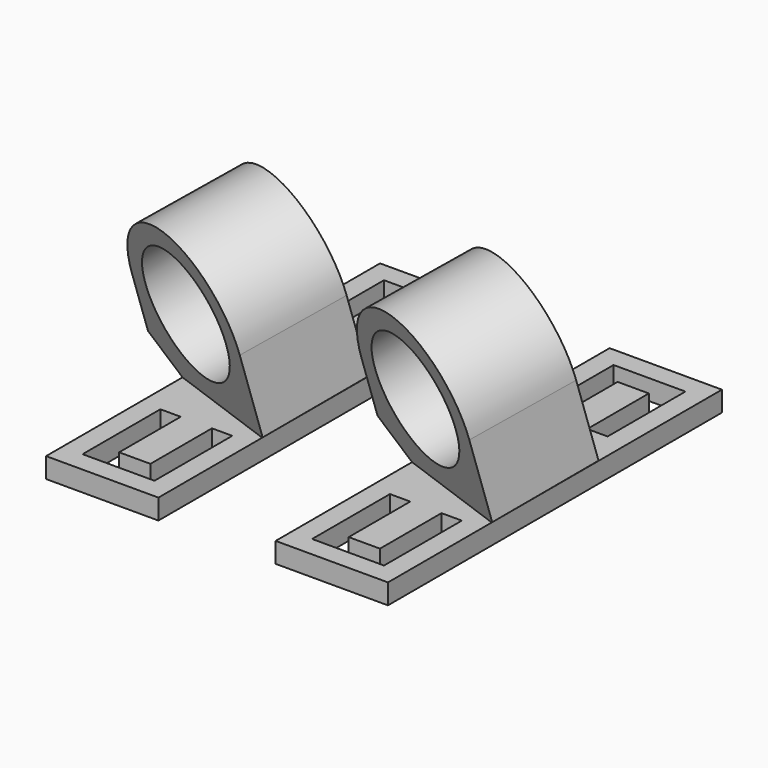
from build123d import *

# Parameters (mm, degrees)
F0_W      = 11.11
F0_H      = 2
F1_DEPTH  = 20.64
F0_R      = 6
F2_DEPTH  = 5
F3_ANGLE  = 15
F4_ANGLE  = -20
F5_REACH  = 31.3423506364
F6_DEPTH  = 6.9
F7_DEPTH  = 25
F11_DEPTH = 25
F12_DEPTH = 31
F15_DEPTH = 25


with BuildPart() as f1:
    # F0 (on Front) → F1 (new body, symmetric)
    with BuildSketch(Plane.XZ):
        with Locations((-58.071229763, 1)):
            Rectangle(F0_W, F0_H)
    extrude(amount=F1_DEPTH, both=True)


with BuildPart() as f2:
    # F0 (on Front) → F2 (new body, symmetric)
    with BuildSketch(Plane.XZ):
        with BuildLine():
            ThreePointArc((-50.071229763, 11.4522753283), (-58.071229763, 19.4522753283), (-66.071229763, 11.4522753283))
            ThreePointArc((-66.071229763, 11.4522753283), (-58.071229763, 3.4522753283), (-50.071229763, 11.4522753283))
        make_face()
        with Locations((-58.071229763, 11.4522753283)):
            Circle(F0_R, mode=Mode.SUBTRACT)
        with BuildLine():
            Line((-66.071229763, 2), (-63.626229763, 2))
            Line((-63.626229763, 2), (-52.516229763, 2))
            Line((-52.516229763, 2), (-50.071229763, 2))
            Line((-50.071229763, 2), (-50.071229763, 11.4522753283))
            ThreePointArc((-50.071229763, 11.4522753283), (-58.071229763, 3.4522753283), (-66.071229763, 11.4522753283))
            Line((-66.071229763, 11.4522753283), (-66.071229763, 2))
        make_face()
    extrude(amount=F2_DEPTH, both=True)


with BuildPart() as f2_1:
    # F3: moved
    add(f2.part.rotate(Axis((-58.071229763, 0, 1), (1, 0, 0)), F3_ANGLE))


with BuildPart() as f2_2:
    # F4: moved
    add(f2_1.part.rotate(Axis((-58.071229763, 0, 1), (0, 0, 1)), F4_ANGLE))


with BuildPart() as f5:
    f5_end = Plane(origin=(-58.071229763, 0, 0), x_dir=(-1, 0, 0), z_dir=(0, 0, -1))
    # F2_face (on face) → F5 (new body, up to a plane its end follows)
    with BuildSketch(Plane(origin=(-58.1597510899, -0.2432103468, 1.9659258263), x_dir=(1, 0, 0), z_dir=(0.0885213269, 0.2432103468, -0.9659258263))):
        Polygon((-9.2055096516, 2.0636356397), (-5.8888283999, -7.3703256425), (9.2055096516, -2.0636356397), (5.8888283999, 7.3703256425), align=None)
    f5_long = extrude(amount=F5_REACH, mode=Mode.PRIVATE)
    add(split(f5_long, bisect_by=f5_end, keep=Keep.BOTTOM, mode=Mode.PRIVATE))


with BuildPart() as f6_tool:
    # F6 (cut): a face of the model
    f6_faces = [f1.part.faces().sort_by_distance(p)[0] for p in [
        (-63.626229763, 0, 1),
    ]]
    extrude(f6_faces, amount=F6_DEPTH)


with BuildPart() as f2_3:
    add(f2_2.part)

    # F6: cut by f6_tool
    add(f6_tool.part, mode=Mode.SUBTRACT)


with BuildPart() as f5_1:
    add(f5.part)

    # F6: cut by f6_tool
    add(f6_tool.part, mode=Mode.SUBTRACT)


with BuildPart() as f7_tool:
    # F7 (cut): a face of the model
    f7_faces = [f1.part.faces().sort_by_distance(p)[0] for p in [
        (-52.516229763, 0, 1),
    ]]
    extrude(f7_faces, amount=F7_DEPTH)


with BuildPart() as f2_4:
    add(f2_3.part)

    # F7: cut by f7_tool
    add(f7_tool.part, mode=Mode.SUBTRACT)


with BuildPart() as f5_2:
    add(f5_1.part)

    # F7: cut by f7_tool
    add(f7_tool.part, mode=Mode.SUBTRACT)


with BuildPart() as f1_1:
    add(f1.part)

    # F8: union F2, F5
    add(f2_4.part)
    add(f5_2.part)


with BuildPart() as f9_1:
    # F9: copy of F1
    add(f1_1.part.moved(Location((28.1, 0, 0))))


with BuildPart() as f1_2:
    add(f1_1.part)

    # F10 (on face) → F11 (cut)
    with BuildSketch(Plane.XZ.offset(20.64)):
        Polygon((-47.5953929126, 6.1317714863), (-52.516229763, 2), (-52.516229763, 0), (-47.5953929126, 0), align=None)
        Polygon((-63.626229763, 0), (-63.626229763, 2), (-68.9108520746, 5.1364828832), (-68.9108520746, 0), align=None)
    extrude(amount=-F11_DEPTH, mode=Mode.SUBTRACT)

    # F10 (on face) → F12 (cut)
    with BuildSketch(Plane.XZ.offset(20.64)):
        Polygon((-47.5953929126, 6.1317714863), (-52.516229763, 2), (-52.516229763, 0), (-47.5953929126, 0), align=None)
        Polygon((-63.626229763, 0), (-63.626229763, 2), (-68.9108520746, 5.1364828832), (-68.9108520746, 0), align=None)
    extrude(amount=-F12_DEPTH, mode=Mode.SUBTRACT)

    # F14 (on face) → F15 (cut)
    with BuildSketch(Plane.XY.offset(2)):
        Polygon((-59.616229763, -9.01), (-61.626229763, -9.01), (-61.626229763, -18.63), (-54.516229763, -18.63), (-54.516229763, -9.01), (-56.526229763, -9.01), (-56.526229763, -16.62), (-59.616229763, -16.62), align=None)
        Polygon((-54.516229763, 18.63), (-61.626229763, 18.63), (-61.626229763, 9.01), (-59.616229763, 9.01), (-59.616229763, 16.62), (-56.526229763, 16.62), (-56.526229763, 9.01), (-54.516229763, 9.01), align=None)
    extrude(amount=-F15_DEPTH, mode=Mode.SUBTRACT)


with BuildPart() as f16_1:
    # F16: copy of F1
    add(f1_2.part.moved(Location((22.7, 0, 0))))


with BuildPart() as f17_1:
    # F17: copy of F1
    add(f1_2.part.moved(Location((43.6, 0, 0))))


solid = Compound([f1_2.part, f16_1.part])
